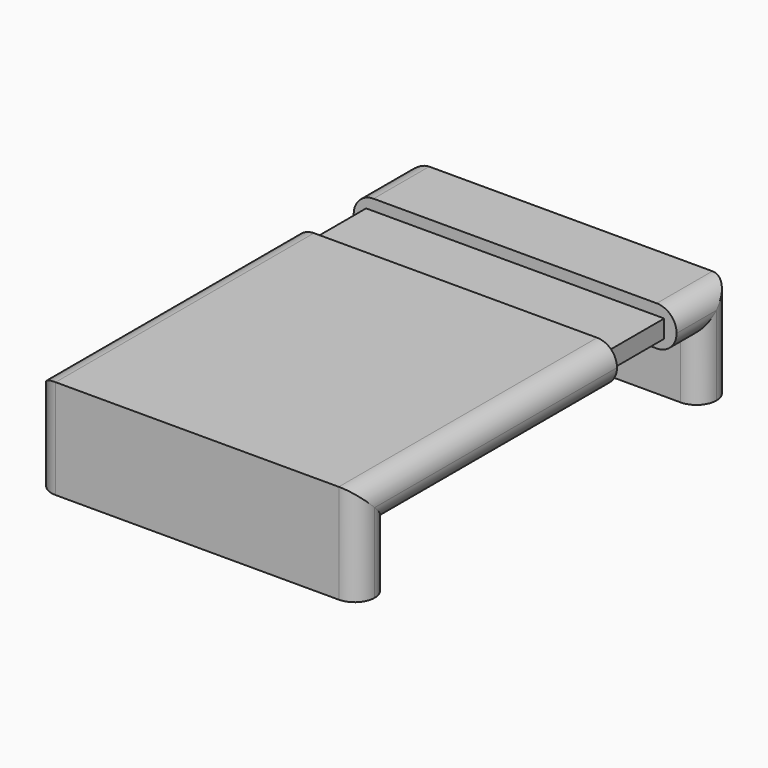
from build123d import *

# Parameters (mm, degrees)
F0_W      = 65
F0_H      = 65
F1_DEPTH  = 8
F2_W      = 65
F2_H      = 20
F3_DEPTH  = 8
F4_W      = 60
F4_H      = 3.6
F5_DEPTH  = 15
F6_R      = 3.99999
F7_W      = 65
F7_H      = 8
F8_DEPTH  = 14
F9_W      = 65
F9_H      = 8
F10_DEPTH = 12
F11_R     = 3.99999


# Not quite as in the source:
# - a fillet or chamfer is up to 0.001 mm smaller than in the source, because OpenCascade refuses the exact size


with BuildPart() as f1:
    # F0 (on Top) → F1 (new body)
    with BuildSketch(Plane.XY):
        Rectangle(F0_W, F0_H)
    extrude(amount=F1_DEPTH)

    # F2 (on face) → F3 (join)
    with BuildSketch(Plane.XZ.offset(32.5)):
        with Locations((0, -2)):
            Rectangle(F2_W, F2_H)
    extrude(amount=-F3_DEPTH)

    # F4 (on face) → F5 (join)
    with BuildSketch(Plane(origin=(0, 32.5, 0), x_dir=(-1, 0, 0), z_dir=(0, 1, 0))):
        with Locations((0, 4)):
            Rectangle(F4_W, F4_H)
    extrude(amount=F5_DEPTH)

    # F6 (radius 4 in the source; OpenCascade refuses exactly that, so slightly less here)
    f6_edges = [f1.edges().sort_by_distance(p)[0] for p in [
        (-32.5, -24.5, -6),
        (-32.5, -32.5, -2),
        (32.5, -24.5, -6),
        (32.5, -32.5, -2),
        (32.5, 0, 8),
        (-32.5, 0, 8),
        (32.5, 4, 0),
        (-32.5, 4, 0),
    ]]
    fillet(f6_edges, radius=F6_R)

    # F7 (on face) → F8 (join)
    with BuildSketch(Plane(origin=(0, 47.5, 0), x_dir=(-1, 0, 0), z_dir=(0, 1, 0))):
        with Locations((0, 4)):
            Rectangle(F7_W, F7_H)
    extrude(amount=F8_DEPTH)

    # F9 (on face) → F10 (join, through all)
    with BuildSketch(Plane(origin=(0, 0, 0), x_dir=(1, 0, 0), z_dir=(0, 0, -1))):
        with Locations((0, -57.5)):
            Rectangle(F9_W, F9_H)
    extrude(amount=F10_DEPTH)

    # F11 (radius 4 in the source; OpenCascade refuses exactly that, so slightly less here)
    f11_edges = [f1.edges().sort_by_distance(p)[0] for p in [
        (-32.5, 61.5, -2),
        (-32.5, 53.5, -6),
        (-32.5, 50.5, 0),
        (-32.5, 54.5, 8),
        (32.5, 50.5, 0),
        (32.5, 54.5, 8),
        (32.5, 61.5, -2),
        (32.5, 53.5, -6),
    ]]
    fillet(f11_edges, radius=F11_R)


solid = f1.part
